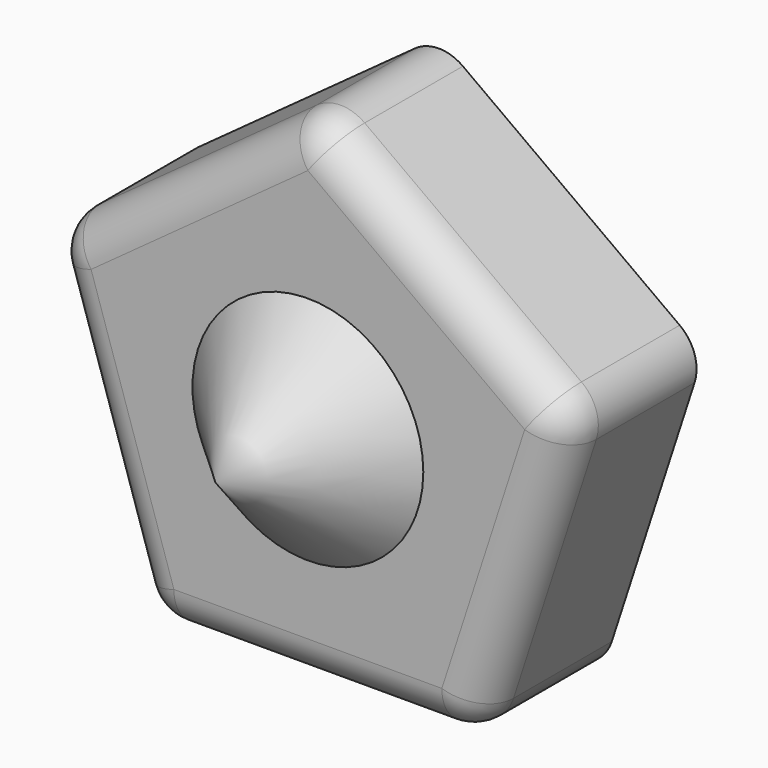
from build123d import *

# Parameters (mm, degrees)
F0_R         = 15
F1_DEPTH     = 20
F2_R         = 5
F3_T1_DEPTH  = 24.0817816001
F3_T6_DEPTH  = 5
F3_T12_DEPTH = 5
F3_T18_DEPTH = 5
F3_T24_DEPTH = 5
F3_T30_DEPTH = 5
F4_DEPTH     = 34.1


# Not quite as in the source:
# - a fillet or chamfer that OpenCascade refuses, or shapes differently, is made with other operations: its cross-section is extruded or revolved along the edge and cut away or added


with BuildPart() as f1:
    # F0 (on Front) → F1 (new body)
    with BuildSketch(Plane.XZ):
        Polygon((-20, -27.5276384094), (20, -27.5276384094), (32.360679775, 10.5146222424), (0, 34.0260323341), (-32.360679775, 10.5146222424), align=None)
        Circle(F0_R, mode=Mode.SUBTRACT)
    extrude(amount=F1_DEPTH)

    # F2
    f2_edges = [f1.edges().sort_by_distance(p)[0] for p in [
        (-26.18034, -20, -8.506508),
        (0, -20, -27.527638),
        (26.18034, -20, -8.506508),
        (16.18034, -20, 22.270327),
        (-16.18034, -20, 22.270327),
    ]]
    fillet(f2_edges, radius=F2_R)

    # F3: fillet of radius 5 on 5 edges, made by hand

    # F3_s2 → F3_t1 (cut)
    with BuildSketch(Plane.XZ.offset(-9.0817816001)):
        with BuildLine():
            ThreePointArc((16.36728736, -27.5276384094), (19.3062136214, -26.5727233813), (21.1225699414, -24.0727233813))
            Line((21.1225699414, -24.0727233813), (20, -27.5276384094))
            Line((20, -27.5276384094), (16.36728736, -27.5276384094))
        make_face()
        with BuildLine():
            ThreePointArc((29.4217535135, 12.649877158), (31.2381098335, 10.149877158), (31.2381098335, 7.0597072143))
            Line((31.2381098335, 7.0597072143), (32.360679775, 10.5146222424))
            Line((32.360679775, 10.5146222424), (29.4217535135, 12.649877158))
        make_face()
        with BuildLine():
            ThreePointArc((-2.9389262615, 31.8907774185), (0, 32.8456924466), (2.9389262615, 31.8907774185))
            Line((2.9389262615, 31.8907774185), (0, 34.0260323341))
            Line((0, 34.0260323341), (-2.9389262615, 31.8907774185))
        make_face()
        with BuildLine():
            ThreePointArc((-31.2381098335, 7.0597072143), (-31.2381098335, 10.149877158), (-29.4217535135, 12.649877158))
            Line((-29.4217535135, 12.649877158), (-32.360679775, 10.5146222424))
            Line((-32.360679775, 10.5146222424), (-31.2381098335, 7.0597072143))
        make_face()
        with BuildLine():
            ThreePointArc((-21.1225699414, -24.0727233813), (-19.3062136214, -26.5727233813), (-16.36728736, -27.5276384094))
            Line((-16.36728736, -27.5276384094), (-20, -27.5276384094))
            Line((-20, -27.5276384094), (-21.1225699414, -24.0727233813))
        make_face()
    extrude(amount=F3_T1_DEPTH, mode=Mode.SUBTRACT)


with BuildPart() as f3_tool4:
    # F3_s5 → F3_t6 (new body)
    with BuildSketch(Plane.XZ.offset(15)):
        Polygon((-16.36728736, -22.5276384094), (-21.1225699414, -24.0727233813), (-20, -27.5276384094), (-16.36728736, -27.5276384094), align=None)
    extrude(amount=F3_T6_DEPTH)

    # F3_s7 → F3_t8 (revolve, cut)
    with BuildSketch(Plane(origin=(-16.36728736, -15, -22.5276384094), x_dir=(0.5877852523, 0, 0.8090169944), z_dir=(0.8090169944, 0, -0.5877852523))):
        with BuildLine():
            ThreePointArc((0, -5), (5, 0), (0, 5))
            Line((0, 5), (0, -5))
        make_face()
    revolve(axis=Axis((-16.36728736, -15, -22.5276384094), (0, -1, 0)), mode=Mode.SUBTRACT)


with BuildPart() as f1_1:
    add(f1.part)

    # F3_t3: cut F3_tool4
    add(f3_tool4.part, mode=Mode.SUBTRACT)


with BuildPart() as f3_tool10:
    # F3_s11 → F3_t12 (new body)
    with BuildSketch(Plane.XZ.offset(15)):
        Polygon((-26.4828272521, 8.6047921861), (-31.2381098335, 7.0597072143), (-32.360679775, 10.5146222424), (-29.4217535135, 12.649877158), align=None)
    extrude(amount=F3_T12_DEPTH)

    # F3_s13 → F3_t14 (revolve, cut)
    with BuildSketch(Plane(origin=(-26.4828272521, -15, 8.6047921861), x_dir=(0.9510565163, 0, -0.3090169944), z_dir=(-0.3090169944, 0, -0.9510565163))):
        with BuildLine():
            ThreePointArc((0, -5), (5, 0), (0, 5))
            Line((0, 5), (0, -5))
        make_face()
    revolve(axis=Axis((-26.4828272521, -15, 8.6047921861), (0, -1, 0)), mode=Mode.SUBTRACT)


with BuildPart() as f1_2:
    add(f1_1.part)

    # F3_t9: cut F3_tool10
    add(f3_tool10.part, mode=Mode.SUBTRACT)


with BuildPart() as f3_tool16:
    # F3_s17 → F3_t18 (new body)
    with BuildSketch(Plane.XZ.offset(15)):
        Polygon((0, 27.8456924466), (-2.9389262615, 31.8907774185), (0, 34.0260323341), (2.9389262615, 31.8907774185), align=None)
    extrude(amount=F3_T18_DEPTH)

    # F3_s19 → F3_t20 (revolve, cut)
    with BuildSketch(Plane(origin=(0, -15, 27.8456924466), x_dir=(0, 0, -1), z_dir=(-1, 0, 0))):
        with BuildLine():
            ThreePointArc((0, -5), (5, 0), (0, 5))
            Line((0, 5), (0, -5))
        make_face()
    revolve(axis=Axis((0, -15, 27.8456924466), (0, -1, 0)), mode=Mode.SUBTRACT)


with BuildPart() as f1_3:
    add(f1_2.part)

    # F3_t15: cut F3_tool16
    add(f3_tool16.part, mode=Mode.SUBTRACT)


with BuildPart() as f3_tool22:
    # F3_s23 → F3_t24 (new body)
    with BuildSketch(Plane.XZ.offset(15)):
        Polygon((26.4828272521, 8.6047921861), (29.4217535135, 12.649877158), (32.360679775, 10.5146222424), (31.2381098335, 7.0597072143), align=None)
    extrude(amount=F3_T24_DEPTH)

    # F3_s25 → F3_t26 (revolve, cut)
    with BuildSketch(Plane(origin=(26.4828272521, -15, 8.6047921861), x_dir=(-0.9510565163, 0, -0.3090169944), z_dir=(-0.3090169944, 0, 0.9510565163))):
        with BuildLine():
            ThreePointArc((0, -5), (5, 0), (0, 5))
            Line((0, 5), (0, -5))
        make_face()
    revolve(axis=Axis((26.4828272521, -15, 8.6047921861), (0, -1, 0)), mode=Mode.SUBTRACT)


with BuildPart() as f1_4:
    add(f1_3.part)

    # F3_t21: cut F3_tool22
    add(f3_tool22.part, mode=Mode.SUBTRACT)


with BuildPart() as f3_tool28:
    # F3_s29 → F3_t30 (new body)
    with BuildSketch(Plane.XZ.offset(15)):
        Polygon((16.36728736, -22.5276384094), (16.36728736, -27.5276384094), (20, -27.5276384094), (21.1225699414, -24.0727233813), align=None)
    extrude(amount=F3_T30_DEPTH)

    # F3_s31 → F3_t32 (revolve, cut)
    with BuildSketch(Plane(origin=(16.36728736, -15, -22.5276384094), x_dir=(-0.5877852523, 0, 0.8090169944), z_dir=(0.8090169944, 0, 0.5877852523))):
        with BuildLine():
            ThreePointArc((0, -5), (5, 0), (0, 5))
            Line((0, 5), (0, -5))
        make_face()
    revolve(axis=Axis((16.36728736, -15, -22.5276384094), (0, -1, 0)), mode=Mode.SUBTRACT)


with BuildPart() as f1_5:
    add(f1_4.part)

    # F3_t27: cut F3_tool28
    add(f3_tool28.part, mode=Mode.SUBTRACT)

    # F0 (on Front) → F4 (join)
    with BuildSketch(Plane.XZ):
        Circle(F0_R)
    extrude(amount=F4_DEPTH)

    # F5: chamfer of 15 on 1 edges, made by hand


with BuildPart() as f5_tool2:
    # F5_s3 → F5_t4 (revolve)
    with BuildSketch(Plane.XY):
        Polygon((15, -19.1), (0, -34.1), (15, -34.1), align=None)
    revolve(axis=Axis((0, -34.1, 0), (0, -1, 0)))

    split(bisect_by=Plane.XZ.offset(20), keep=Keep.TOP)


with BuildPart() as f1_6:
    add(f1_5.part)

    # F5_t1: cut F5_tool2
    add(f5_tool2.part, mode=Mode.SUBTRACT)


solid = f1_6.part
